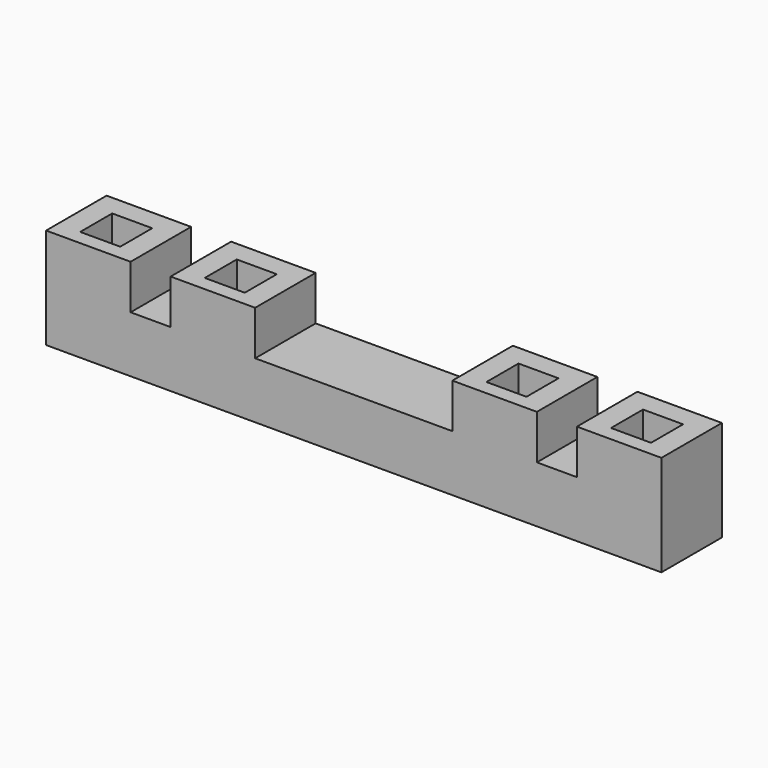
from build123d import *

# Parameters (mm, degrees)
F0_W     = 83
F0_H     = 7.6
F0_W_2   = 79.5
F0_H_2   = 2.6
F1_DEPTH = 7
F2_W     = 83
F2_H     = 7.6
F2_W_2   = 79.5
F2_H_2   = 2.6
F3_DEPTH = 3.2
F4_W     = 3
F4_H     = 2
F4_W_2   = 5.4
F4_H_2   = 5.4
F4_H_3   = 2.8
F5_DEPTH = 6


with BuildPart() as f1:
    # F0 (on Front) → F1 (new body)
    with BuildSketch(Plane.XZ):
        Rectangle(F0_W, F0_H)
        Rectangle(F0_W_2, F0_H_2, mode=Mode.SUBTRACT)
    extrude(amount=F1_DEPTH)

    # F2 (on face) → F3 (join)
    with BuildSketch(Plane.XZ.offset(7)):
        Rectangle(F2_W, F2_H)
        Rectangle(F2_W_2, F2_H_2, mode=Mode.SUBTRACT)
        Rectangle(F2_W_2, F2_H_2)
    extrude(amount=F3_DEPTH)

    # F4 (on face) → F5 (join)
    with BuildSketch(Plane.XY.offset(3.8)):
        with Locations((-40, -9.2)):
            Rectangle(F4_W, F4_H)
        with Locations((-35.8, -9.2)):
            Rectangle(F4_W_2, F4_H)
        with Locations((-40, -5.5)):
            Rectangle(F4_W, F4_H_2)
        with Locations((-31.6, -9.2)):
            Rectangle(F4_W, F4_H)
        with Locations((-40, -1.4)):
            Rectangle(F4_W, F4_H_3)
        with Locations((-31.6, -5.5)):
            Rectangle(F4_W, F4_H_2)
        with Locations((-35.8, -1.4)):
            Rectangle(F4_W_2, F4_H_3)
        with Locations((-23.2, -9.2)):
            Rectangle(F4_W, F4_H)
        with Locations((-31.6, -1.4)):
            Rectangle(F4_W, F4_H_3)
        with Locations((-19, -9.2)):
            Rectangle(F4_W_2, F4_H)
        with Locations((-23.2, -5.5)):
            Rectangle(F4_W, F4_H_2)
        with Locations((-14.8, -9.2)):
            Rectangle(F4_W, F4_H)
        with Locations((-23.2, -1.4)):
            Rectangle(F4_W, F4_H_3)
        with Locations((-14.8, -5.5)):
            Rectangle(F4_W, F4_H_2)
        with Locations((-19, -1.4)):
            Rectangle(F4_W_2, F4_H_3)
        with Locations((-14.8, -1.4)):
            Rectangle(F4_W, F4_H_3)
        with Locations((14.8, -9.2)):
            Rectangle(F4_W, F4_H)
        with Locations((19, -9.2)):
            Rectangle(F4_W_2, F4_H)
        with Locations((14.8, -5.5)):
            Rectangle(F4_W, F4_H_2)
        with Locations((23.2, -9.2)):
            Rectangle(F4_W, F4_H)
        with Locations((14.8, -1.4)):
            Rectangle(F4_W, F4_H_3)
        with Locations((23.2, -5.5)):
            Rectangle(F4_W, F4_H_2)
        with Locations((19, -1.4)):
            Rectangle(F4_W_2, F4_H_3)
        with Locations((31.6, -9.2)):
            Rectangle(F4_W, F4_H)
        with Locations((23.2, -1.4)):
            Rectangle(F4_W, F4_H_3)
        with Locations((35.8, -9.2)):
            Rectangle(F4_W_2, F4_H)
        with Locations((31.6, -5.5)):
            Rectangle(F4_W, F4_H_2)
        with Locations((40, -9.2)):
            Rectangle(F4_W, F4_H)
        with Locations((31.6, -1.4)):
            Rectangle(F4_W, F4_H_3)
        with Locations((40, -5.5)):
            Rectangle(F4_W, F4_H_2)
        with Locations((35.8, -1.4)):
            Rectangle(F4_W_2, F4_H_3)
        with Locations((40, -1.4)):
            Rectangle(F4_W, F4_H_3)
    extrude(amount=F5_DEPTH)


solid = f1.part
